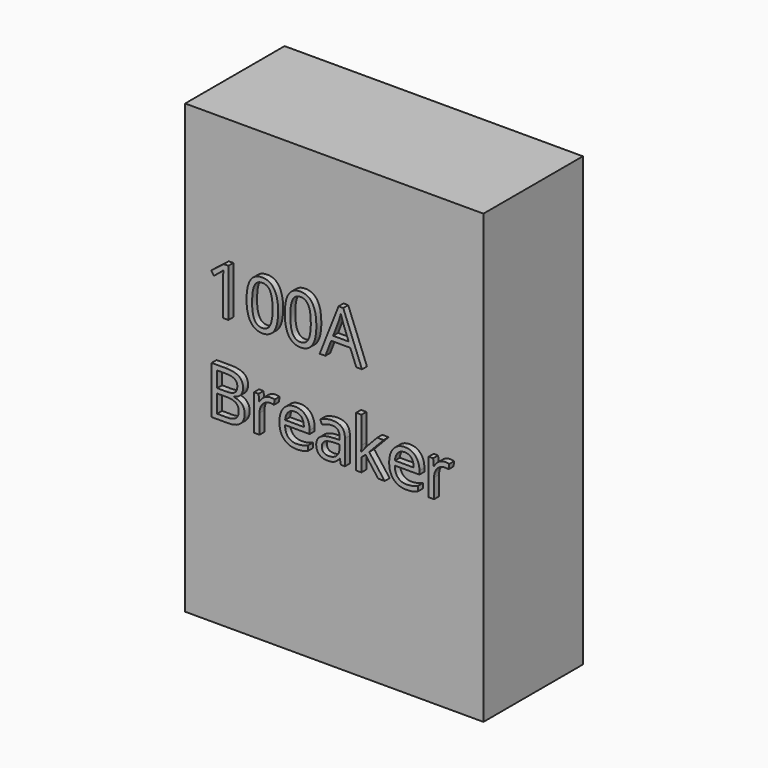
from build123d import *

# Parameters (mm, degrees)
F0_W         = 609.6
F0_H         = 914.4
F1_DEPTH     = 254
F2_TEXT_SIZE = 136.6222633105
F3_DEPTH     = 12.7


# Not quite as in the source:
# - Text() gives the source's letters only with a copy of the font that has no kerning and outlines rounded to 1/6400 em; it was checked with that copy


with BuildPart() as f1:
    # F0 (on Front) → F1 (new body)
    with BuildSketch(Plane.XZ):
        Rectangle(F0_W, F0_H)
    extrude(amount=F1_DEPTH)

    # F2 (on face) → F3 (join)
    with BuildSketch(Plane.XZ.offset(254)):
        with Locations((-254, 104.8319704164)):
            Text('100A', F2_TEXT_SIZE, font='Open Sans', text_align=(TextAlign.LEFT, TextAlign.BOTTOM))
        with Locations((-254, -80.9743076858)):
            Text('Breaker', F2_TEXT_SIZE, font='Open Sans', text_align=(TextAlign.LEFT, TextAlign.BOTTOM))
    extrude(amount=F3_DEPTH)


solid = f1.part
